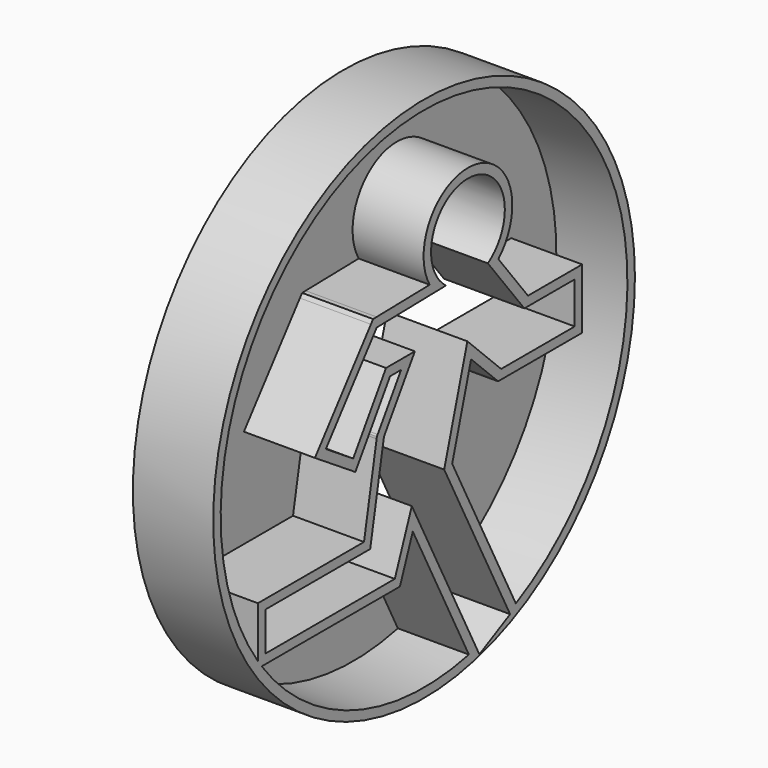
from build123d import *

# Parameters (mm, degrees)
F0_R        = 71.6651662247
F1_DEPTH    = 21.844
F2_T        = 2.54
F2_T3_DEPTH = 26.924


# Not quite as in the source:
# - a shell that OpenCascade refuses in one call is made with other operations: the cavity is built on its own and cut out
# - a feature names something its author has since deleted; it is built from what else it names


with BuildPart() as f1:
    # F0 (on Right) → F1 (new body)
    with BuildSketch(Plane.YZ):
        with Locations((-115.809135139, -7.7714063227)):
            Circle(F0_R)
        with BuildLine():
            ThreePointArc((-108.3759665489, 16.3117386401), (-100.4681563218, 38.9034837812), (-94.1200479865, 15.824880451))
            Line((-94.1200479865, 15.824880451), (-81.7305743694, 0))
            Line((-81.7305743694, 0), (-64.600661397, 0))
            Line((-64.600661397, 0), (-64.600661397, -11.2849194556))
            Line((-64.600661397, -11.2849194556), (-89.6177664399, -11.2849194556))
            Line((-89.6177664399, -11.2849194556), (-101.0896414518, 0))
            Line((-101.0896414518, 0), (-108.967371285, -27.4995788932))
            Line((-108.967371285, -27.4995788932), (-86.5627974272, -71.233086288))
            Line((-86.5627974272, -71.233086288), (-97.011906829, -76.5861406686))
            Line((-97.011906829, -76.5861406686), (-119.9753677787, -31.7616911776))
            Line((-119.9753677787, -31.7616911776), (-125.7533729076, -46.8470752239))
            Line((-125.7533729076, -46.8470752239), (-152.9145538807, -46.8470752239))
            Line((-152.9145538807, -46.8470752239), (-156.1464071274, -46.8470752239))
            Line((-156.1464071274, -46.8470752239), (-169.7414368391, -46.8470752239))
            Line((-169.7414368391, -46.8470752239), (-169.7414368391, -36.2966917455))
            Line((-169.7414368391, -36.2966917455), (-156.1464071274, -36.2966917455))
            Line((-156.1464071274, -36.2966917455), (-134.1130137444, -36.2966917455))
            Line((-134.1130137444, -36.2966917455), (-129.4415742159, -11.2849194556))
            Line((-129.4415742159, -11.2849194556), (-118.9312636852, 4.8525910825))
            Line((-118.9312636852, 4.8525910825), (-128.7393420935, 4.8525910825))
            Line((-128.7393420935, 4.8525910825), (-139.9055675141, -12.2920099139))
            Line((-139.9055675141, -12.2920099139), (-149.2000942902, -6.2385134702))
            Line((-149.2000942902, -6.2385134702), (-131.8777501583, 15.824880451))
            Line((-131.8777501583, 15.824880451), (-108.3759665489, 16.3117386401))
        make_face(mode=Mode.SUBTRACT)
    extrude(amount=F1_DEPTH)

    # F2: shell of thickness 2.54, made by hand


with BuildPart() as f2_core1:
    # F2_t2: copy of F1
    add(f1.part)

    # the walls: a layer under each face that stays
    f2_faces = [f2_core1.faces().sort_by_distance(p)[0] for p in [
        (10.922, -187.4743013637, -7.7714063227),
        (10.922, -140.5389222243, 4.7931834904),
        (10.922, -144.5528309022, -9.2652616921),
        (10.922, -134.3224548038, -3.7197094157),
        (10.922, -123.8353028893, 4.8525910825),
        (10.922, -124.1864189506, -3.2161641866),
        (10.922, -131.7772939801, -23.7908056006),
        (10.922, -151.9272252917, -36.2966917455),
        (10.922, -169.7414368391, -41.5718834847),
        (10.922, -147.7474048734, -46.8470752239),
        (10.922, -122.8643703432, -39.3043832007),
        (10.922, -108.4936373039, -54.1739159231),
        (10.922, -91.7873521281, -73.9096134783),
        (10.922, -97.7650843561, -49.3663325906),
        (10.922, -105.0285063684, -13.7497894466),
        (10.922, -95.3537039459, -5.6424597278),
        (10.922, -77.1092139184, -11.2849194556),
        (10.922, -64.600661397, -5.6424597278),
        (10.922, -73.1656178832, 0),
        (10.922, -87.925311178, 7.9124402255),
        (10.922, -100.4681563218, 38.9034837812),
        (10.922, -120.1268583536, 16.0683095455),
        (0, -163.5859126221, -55.5481838059),
    ]]
    thicken(f2_faces, amount=-F2_T, mode=Mode.SUBTRACT)

    # F2_s4 → F2_t3 (cut)
    with BuildSketch(Plane.YZ.offset(-2.54)):
        Polygon((-149.1662539052, -6.2329149117), (-151.197922499, -4.6699847175), (-152.9114712381, -6.8525242483), (-150.5863045792, -8.3668980771), align=None)
        Polygon((-131.8572458078, 15.7838006118), (-133.8755783671, 17.3934092037), (-133.1328452619, 18.3394251098), (-131.9303569971, 18.3643356131), align=None)
        Polygon((-139.9129892573, -12.256863965), (-141.2917778031, -14.4203945208), (-139.1633931962, -15.8066048098), (-137.7771829073, -13.6782202029), align=None)
        Polygon((-129.3953221194, -11.3034448695), (-131.5699588227, -9.8987091667), (-131.8456535688, -10.3220103485), (-131.9383992614, -10.8185883585), align=None)
        Polygon((-169.7160368391, -36.3220917455), (-169.7414368391, -33.7566917455), (-172.2814368391, -33.7566917455), (-172.2814368391, -36.2966917455), align=None)
        Polygon((-169.7160368391, -46.8216752239), (-172.2814368391, -46.8470752239), (-172.2814368391, -49.3870752239), (-169.7414368391, -49.3870752239), align=None)
        Polygon((-125.7770925414, -46.8125901277), (-125.7533729076, -49.3870752239), (-124.0063031182, -49.3870752239), (-123.3814095297, -47.7555848463), align=None)
        Polygon((-97.0008817516, -76.5519534244), (-99.2725229084, -77.7442490147), (-98.1144145624, -80.0048650942), (-95.8537984829, -78.8467567481), align=None)
        Polygon((-86.5969846714, -71.2220612106), (-85.4046890811, -73.4937023674), (-83.1440730016, -72.3355940214), (-84.3021813477, -70.0749779419), align=None)
        Polygon((-89.5999540811, -11.2414120021), (-91.3990023244, -13.095664806), (-90.6576662231, -13.8249194556), (-89.6177664399, -13.8249194556), align=None)
        Polygon((-64.626061397, -11.2595194556), (-64.600661397, -13.8249194556), (-62.060661397, -13.8249194556), (-62.060661397, -11.2849194556), align=None)
        Polygon((-64.626061397, -0.0254), (-62.060661397, 0), (-62.060661397, 2.54), (-64.600661397, 2.54), align=None)
    extrude(amount=F2_T3_DEPTH, mode=Mode.SUBTRACT)


with BuildPart() as f1_1:
    add(f1.part)

    # what is left inside the walls is the cavity
    f2_cavity = [f2_core1.part.solids().sort_by_distance(p)[0] for p in [
        (15.409333, -139.586841, -72.651283),
        (21.8186, -150.371718, 17.74945),
    ]]
    add(f2_cavity, mode=Mode.SUBTRACT)


solid = f1_1.part
